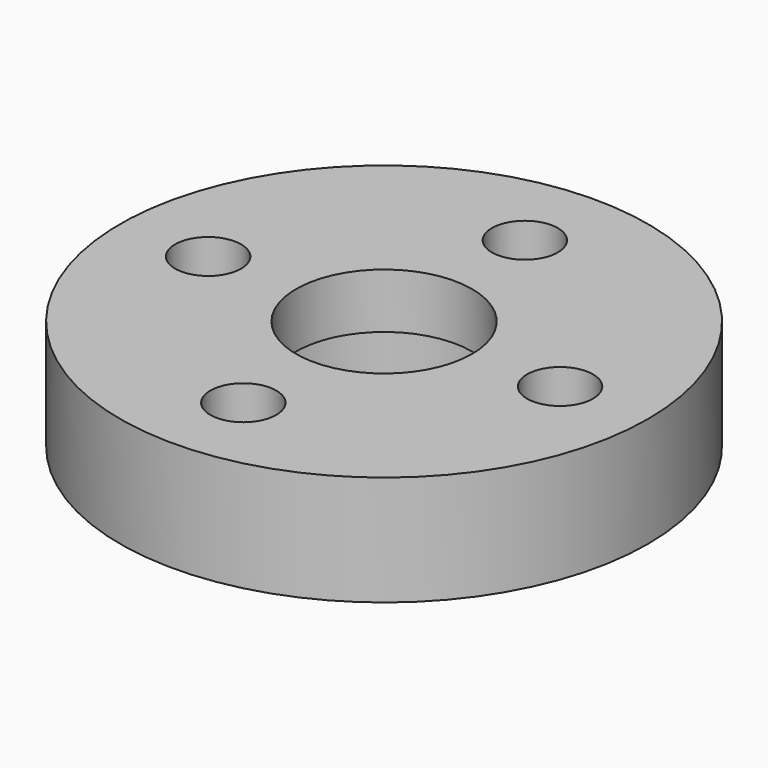
from build123d import *

# Parameters (mm, degrees)
F0_R            = 12
F1_DEPTH        = 5
F2_R            = 4
F3_DEPTH        = 5
F5_R            = 1.5
F6_DEPTH        = 5
F6_COPIES_COUNT = 4
F4_R            = 5.25
F7_DEPTH        = 2.5


# Not quite as in the source:
# - a pattern or mirror of a feature is missing from the dataset's text; its kind, count and spacing are read off the source's solid


with BuildPart() as f1:
    # F0 (on Top) → F1 (new body)
    with BuildSketch(Plane.XY):
        Circle(F0_R)
    extrude(amount=F1_DEPTH)

    # F2 (on face) → F3 (cut, through all)
    with BuildSketch(Plane(origin=(0, 0, 0), x_dir=(1, 0, 0), z_dir=(0, 0, -1))):
        Circle(F2_R)
    extrude(amount=-F3_DEPTH, mode=Mode.SUBTRACT)

    # F5 (on face) → F6 (cut, through all)
    with BuildSketch(Plane(origin=(0, 0, 0), x_dir=(1, 0, 0), z_dir=(0, 0, -1))):
        with Locations((-8, 0)):
            Circle(F5_R)
    f6 = extrude(amount=-F6_DEPTH, mode=Mode.SUBTRACT)

    # F6_copies: F6 ×4 about axis
    f6_copies_axis = Axis((0, 0, 0), (0, 0, 1))
    for i in range(1, F6_COPIES_COUNT):
        add(f6.rotate(f6_copies_axis, i * 360 / F6_COPIES_COUNT), mode=Mode.SUBTRACT)

    # F4 (on face) → F7 (cut)
    with BuildSketch(Plane(origin=(0, 0, 0), x_dir=(1, 0, 0), z_dir=(0, 0, -1))):
        Circle(F4_R)
    extrude(amount=-F7_DEPTH, mode=Mode.SUBTRACT)


solid = f1.part
